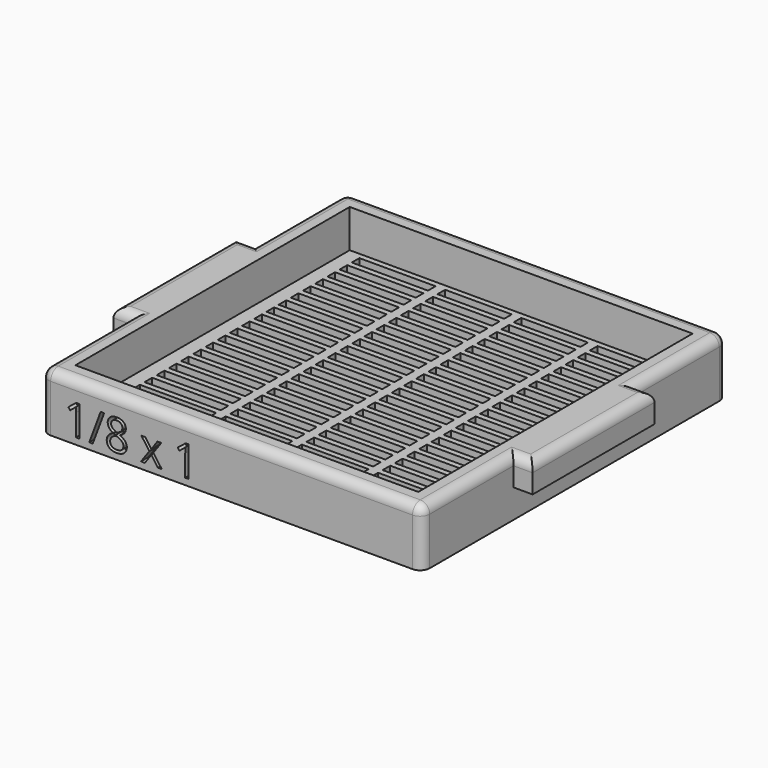
from build123d import *

# Parameters (mm, degrees)
F1_DEPTH     = 6.35
F0_W         = 6.35
F0_H         = 50.8
F2_DEPTH     = 19.05
F3_W         = 25.4
F3_H         = 3.175
F3_W_2       = 22.225
F4_DEPTH     = 25.4
F5_R         = 3.175
F6_W         = 6.35
F6_H         = 50.8
F7_DEPTH     = 9.525
F8_TEXT_SIZE = 14.2674456583
F9_DEPTH     = 3.175


# Not quite as in the source:
# - Text() gives the source's letters only with a copy of the font that has no kerning and outlines rounded to 1/6400 em; it was checked with that copy


with BuildPart() as f1:
    # F0 (on Top) → F1 (new body)
    with BuildSketch(Plane.XY):
        Polygon((-57.15, 25.1415750563), (-57.15, -25.6584249437), (-57.15, -57.4084249437), (57.15, -57.4084249437), (57.15, -25.6584249437), (57.15, 25.1415750563), (57.15, 56.8915750563), (-57.15, 56.8915750563), align=None)
    extrude(amount=F1_DEPTH)

    # F0 (on Top) → F2 (join)
    with BuildSketch(Plane.XY):
        Polygon((-63.5, -25.6584249437), (-63.5, -63.7584249437), (63.5, -63.7584249437), (63.5, -25.6584249437), (57.15, -25.6584249437), (57.15, -57.4084249437), (-57.15, -57.4084249437), (-57.15, -25.6584249437), align=None)
        with Locations((-66.675, -0.2584249437)):
            Rectangle(F0_W, F0_H)
        with Locations((-60.325, -0.2584249437)):
            Rectangle(F0_W, F0_H)
        with Locations((60.325, -0.2584249437)):
            Rectangle(F0_W, F0_H)
        with Locations((66.675, -0.2584249437)):
            Rectangle(F0_W, F0_H)
        Polygon((-63.5, 63.2415750563), (-63.5, 25.1415750563), (-57.15, 25.1415750563), (-57.15, 56.8915750563), (57.15, 56.8915750563), (57.15, 25.1415750563), (63.5, 25.1415750563), (63.5, 63.2415750563), align=None)
    extrude(amount=F2_DEPTH)

    # F3 (on face) → F4 (cut)
    with BuildSketch(Plane.XY.offset(6.35)):
        with Locations((-39.7002, -53.2809249437)):
            Rectangle(F3_W, F3_H)
        with Locations((-39.7002, -48.2009249437)):
            Rectangle(F3_W, F3_H)
        with Locations((-39.7002, -43.1209249437)):
            Rectangle(F3_W, F3_H)
        with Locations((-39.7002, -38.0409249437)):
            Rectangle(F3_W, F3_H)
        with Locations((-39.7002, -32.9609249437)):
            Rectangle(F3_W, F3_H)
        with Locations((-39.7002, -27.8809249437)):
            Rectangle(F3_W, F3_H)
        with Locations((-39.7002, -22.8009249437)):
            Rectangle(F3_W, F3_H)
        with Locations((-39.7002, -17.7209249437)):
            Rectangle(F3_W, F3_H)
        with Locations((-39.7002, -12.6409249437)):
            Rectangle(F3_W, F3_H)
        with Locations((-39.7002, -7.5609249437)):
            Rectangle(F3_W, F3_H)
        with Locations((-39.7002, -2.4809249437)):
            Rectangle(F3_W, F3_H)
        with Locations((-39.7002, 2.5990750563)):
            Rectangle(F3_W, F3_H)
        with Locations((-39.7002, 7.6790750563)):
            Rectangle(F3_W, F3_H)
        with Locations((-39.7002, 12.7590750563)):
            Rectangle(F3_W, F3_H)
        with Locations((-39.7002, 17.8390750563)):
            Rectangle(F3_W, F3_H)
        with Locations((-39.7002, 22.9190750563)):
            Rectangle(F3_W, F3_H)
        with Locations((-39.7002, 27.9990750563)):
            Rectangle(F3_W, F3_H)
        with Locations((-39.7002, 33.0790750563)):
            Rectangle(F3_W, F3_H)
        with Locations((-39.7002, 38.1590750563)):
            Rectangle(F3_W, F3_H)
        with Locations((-39.7002, 43.2390750563)):
            Rectangle(F3_W, F3_H)
        with Locations((-39.7002, 48.3190750563)):
            Rectangle(F3_W, F3_H)
        with Locations((-39.7002, 53.3990750563)):
            Rectangle(F3_W, F3_H)
        with Locations((-12.7127, -53.2809249437)):
            Rectangle(F3_W_2, F3_H)
        with Locations((-12.7127, -48.2009249437)):
            Rectangle(F3_W_2, F3_H)
        with Locations((12.6873, -53.2809249437)):
            Rectangle(F3_W_2, F3_H)
        with Locations((12.6873, -48.2009249437)):
            Rectangle(F3_W_2, F3_H)
        with Locations((39.6748, -53.2809249437)):
            Rectangle(F3_W, F3_H)
        with Locations((39.6748, -48.2009249437)):
            Rectangle(F3_W, F3_H)
        with Locations((39.6748, -43.1209249437)):
            Rectangle(F3_W, F3_H)
        with Locations((39.6748, -38.0409249437)):
            Rectangle(F3_W, F3_H)
        with Locations((12.6873, -38.0409249437)):
            Rectangle(F3_W_2, F3_H)
        with Locations((12.6873, -43.1209249437)):
            Rectangle(F3_W_2, F3_H)
        with Locations((-12.7127, -43.1209249437)):
            Rectangle(F3_W_2, F3_H)
        with Locations((-12.7127, -38.0409249437)):
            Rectangle(F3_W_2, F3_H)
        with Locations((39.6748, -32.9609249437)):
            Rectangle(F3_W, F3_H)
        with Locations((39.6748, -27.8809249437)):
            Rectangle(F3_W, F3_H)
        with Locations((39.6748, -22.8009249437)):
            Rectangle(F3_W, F3_H)
        with Locations((12.6873, -32.9609249437)):
            Rectangle(F3_W_2, F3_H)
        with Locations((12.6873, -27.8809249437)):
            Rectangle(F3_W_2, F3_H)
        with Locations((12.6873, -22.8009249437)):
            Rectangle(F3_W_2, F3_H)
        with Locations((-12.7127, -32.9609249437)):
            Rectangle(F3_W_2, F3_H)
        with Locations((-12.7127, -27.8809249437)):
            Rectangle(F3_W_2, F3_H)
        with Locations((-12.7127, -22.8009249437)):
            Rectangle(F3_W_2, F3_H)
        with Locations((-12.7127, -17.7209249437)):
            Rectangle(F3_W_2, F3_H)
        with Locations((-12.7127, -12.6409249437)):
            Rectangle(F3_W_2, F3_H)
        with Locations((-12.7127, -7.5609249437)):
            Rectangle(F3_W_2, F3_H)
        with Locations((-12.7127, -2.4809249437)):
            Rectangle(F3_W_2, F3_H)
        with Locations((12.6873, -17.7209249437)):
            Rectangle(F3_W_2, F3_H)
        with Locations((12.6873, -12.6409249437)):
            Rectangle(F3_W_2, F3_H)
        with Locations((12.6873, -7.5609249437)):
            Rectangle(F3_W_2, F3_H)
        with Locations((12.6873, -2.4809249437)):
            Rectangle(F3_W_2, F3_H)
        with Locations((39.6748, -2.4809249437)):
            Rectangle(F3_W, F3_H)
        with Locations((39.6748, -7.5609249437)):
            Rectangle(F3_W, F3_H)
        with Locations((39.6748, -12.6409249437)):
            Rectangle(F3_W, F3_H)
        with Locations((39.6748, -17.7209249437)):
            Rectangle(F3_W, F3_H)
        with Locations((-12.7127, 2.5990750563)):
            Rectangle(F3_W_2, F3_H)
        with Locations((-12.7127, 7.6790750563)):
            Rectangle(F3_W_2, F3_H)
        with Locations((-12.7127, 12.7590750563)):
            Rectangle(F3_W_2, F3_H)
        with Locations((-12.7127, 17.8390750563)):
            Rectangle(F3_W_2, F3_H)
        with Locations((-12.7127, 22.9190750563)):
            Rectangle(F3_W_2, F3_H)
        with Locations((-12.7127, 27.9990750563)):
            Rectangle(F3_W_2, F3_H)
        with Locations((-12.7127, 33.0790750563)):
            Rectangle(F3_W_2, F3_H)
        with Locations((-12.7127, 38.1590750563)):
            Rectangle(F3_W_2, F3_H)
        with Locations((-12.7127, 43.2390750563)):
            Rectangle(F3_W_2, F3_H)
        with Locations((-12.7127, 48.3190750563)):
            Rectangle(F3_W_2, F3_H)
        with Locations((-12.7127, 53.3990750563)):
            Rectangle(F3_W_2, F3_H)
        with Locations((12.6873, 53.3990750563)):
            Rectangle(F3_W_2, F3_H)
        with Locations((12.6873, 48.3190750563)):
            Rectangle(F3_W_2, F3_H)
        with Locations((12.6873, 43.2390750563)):
            Rectangle(F3_W_2, F3_H)
        with Locations((12.6873, 38.1590750563)):
            Rectangle(F3_W_2, F3_H)
        with Locations((12.6873, 33.0790750563)):
            Rectangle(F3_W_2, F3_H)
        with Locations((12.6873, 27.9990750563)):
            Rectangle(F3_W_2, F3_H)
        with Locations((12.6873, 22.9190750563)):
            Rectangle(F3_W_2, F3_H)
        with Locations((12.6873, 17.8390750563)):
            Rectangle(F3_W_2, F3_H)
        with Locations((12.6873, 12.7590750563)):
            Rectangle(F3_W_2, F3_H)
        with Locations((12.6873, 7.6790750563)):
            Rectangle(F3_W_2, F3_H)
        with Locations((12.6873, 2.5990750563)):
            Rectangle(F3_W_2, F3_H)
        with Locations((39.6748, 2.5990750563)):
            Rectangle(F3_W, F3_H)
        with Locations((39.6748, 7.6790750563)):
            Rectangle(F3_W, F3_H)
        with Locations((39.6748, 12.7590750563)):
            Rectangle(F3_W, F3_H)
        with Locations((39.6748, 17.8390750563)):
            Rectangle(F3_W, F3_H)
        with Locations((39.6748, 22.9190750563)):
            Rectangle(F3_W, F3_H)
        with Locations((39.6748, 27.9990750563)):
            Rectangle(F3_W, F3_H)
        with Locations((39.6748, 33.0790750563)):
            Rectangle(F3_W, F3_H)
        with Locations((39.6748, 38.1590750563)):
            Rectangle(F3_W, F3_H)
        with Locations((39.6748, 43.2390750563)):
            Rectangle(F3_W, F3_H)
        with Locations((39.6748, 48.3190750563)):
            Rectangle(F3_W, F3_H)
        with Locations((39.6748, 53.3990750563)):
            Rectangle(F3_W, F3_H)
    extrude(amount=-F4_DEPTH, mode=Mode.SUBTRACT)

    # F5
    f5_edges = [f1.edges().sort_by_distance(p)[0] for p in [
        (-63.5, -44.708425, 19.05),
        (0, -63.758425, 19.05),
        (63.5, -44.708425, 19.05),
        (66.675, -25.658425, 19.05),
        (69.85, -0.258425, 19.05),
        (-66.675, -25.658425, 19.05),
        (-69.85, -0.258425, 19.05),
        (-66.675, 25.141575, 19.05),
        (-63.5, 44.191575, 19.05),
        (0, 63.241575, 19.05),
        (63.5, 44.191575, 19.05),
        (66.675, 25.141575, 19.05),
        (63.5, -63.758425, 9.525),
        (-63.5, -63.758425, 9.525),
        (-63.5, 63.241575, 9.525),
        (63.5, 63.241575, 9.525),
    ]]
    fillet(f5_edges, radius=F5_R)

    # F6 (on face) → F7 (cut)
    with BuildSketch(Plane(origin=(0, 0, 0), x_dir=(1, 0, 0), z_dir=(0, 0, -1))):
        with Locations((-66.675, 0.2584249437)):
            Rectangle(F6_W, F6_H)
        with Locations((66.675, 0.2584249437)):
            Rectangle(F6_W, F6_H)
    extrude(amount=-F7_DEPTH, mode=Mode.SUBTRACT)

    # F8 (on face) → F9 (cut)
    with BuildSketch(Plane.XZ.offset(63.7584249437)):
        with Locations((-55.7500422001, 2.1591845434)):
            Text('1/8 x 1', F8_TEXT_SIZE, font='Open Sans', text_align=(TextAlign.LEFT, TextAlign.BOTTOM))
    extrude(amount=-F9_DEPTH, mode=Mode.SUBTRACT)


solid = f1.part
